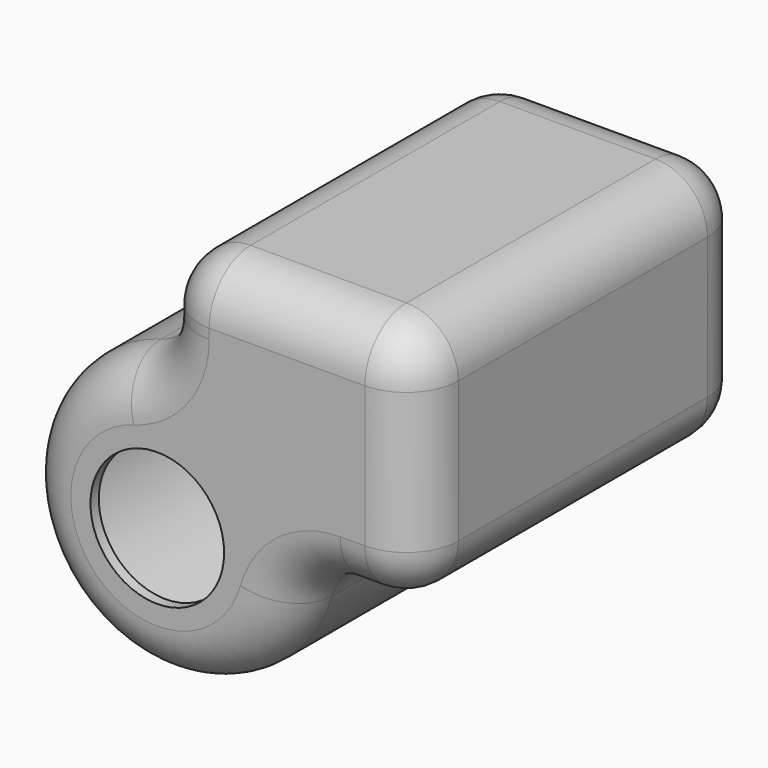
from build123d import *

# Parameters (mm, degrees)
F1_DEPTH = 101.6
F2_R     = 12.7
F3_R     = 16.353641652
F4_DEPTH = 101.601
F5_T     = -2.54


with BuildPart() as f1:
    # F0 (on Front) → F1 (new body)
    with BuildSketch(Plane.XZ):
        with BuildLine():
            ThreePointArc((0, 33.8403694774), (-23.9287547353, -23.9287547353), (33.8403694774, 0))
            Line((33.8403694774, 0), (63.5, 0))
            Line((63.5, 0), (63.5, 59.877499095))
            Line((63.5, 59.877499095), (0, 59.877499095))
            Line((0, 59.877499095), (0, 33.8403694774))
        make_face()
    extrude(amount=F1_DEPTH)

    # F2
    f2_edges = [f1.edges().sort_by_distance(p)[0] for p in [
        (63.5, -50.8, 59.877499),
        (33.840369, -50.8, 0),
        (63.5, -50.8, 0),
        (48.670185, 0, 0),
        (48.670185, -101.6, 0),
        (63.5, -101.6, 29.93875),
        (-23.928755, -101.6, -23.928755),
        (31.75, -101.6, 59.877499),
        (0, -101.6, 46.858934),
        (63.5, 0, 29.93875),
        (31.75, 0, 59.877499),
        (0, -50.8, 59.877499),
        (0, 0, 46.858934),
        (0, -50.8, 33.840369),
        (-23.928755, 0, -23.928755),
    ]]
    fillet(f2_edges, radius=F2_R)

    # F3 (on face) → F4 (cut, through all)
    with BuildSketch(Plane.XZ.offset(101.6)):
        Circle(F3_R)
    extrude(amount=-F4_DEPTH, mode=Mode.SUBTRACT)

    # F5
    f5_openings = [f1.faces().sort_by_distance(p)[0] for p in [
        (-16.353642, -50.8, 0),
    ]]
    offset(amount=F5_T, openings=f5_openings)


solid = f1.part
